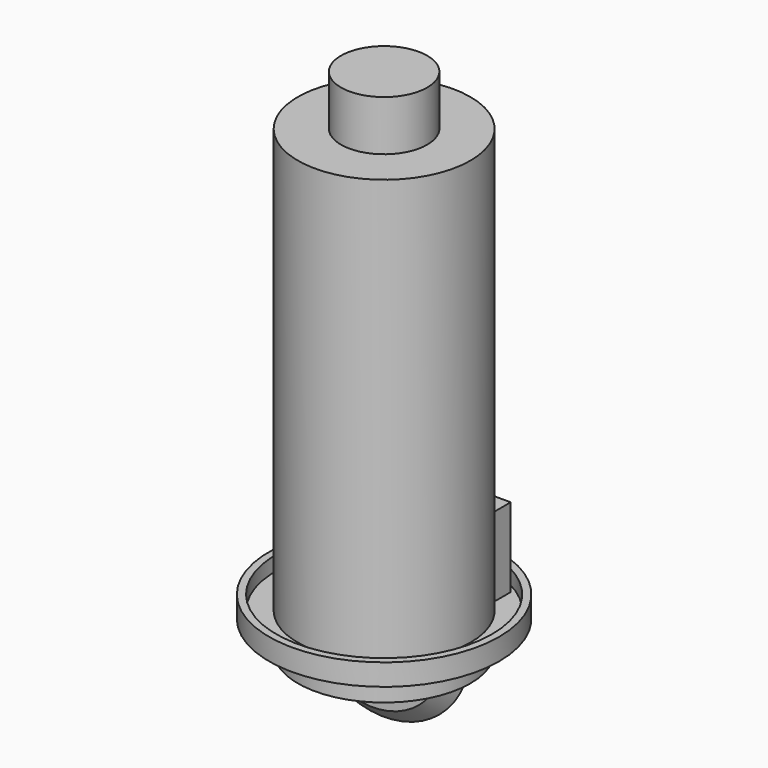
from build123d import *

# Parameters (mm, degrees)
F1_DEPTH  = 76.2
F2_R      = 76.2
F3_DEPTH  = 12.7
F4_SIZE   = 12.69999
F5_R      = 76.2
F5_R_2    = 69.85
F6_DEPTH  = 355.6
F7_R      = 76.2
F8_DEPTH  = 25.4
F9_R      = 76.2
F9_R_2    = 38.1
F10_DEPTH = 25.4
F11_R     = 101.6
F12_DEPTH = 6.35
F13_R     = 101.6
F13_R_2   = 95.25
F14_DEPTH = 12.7
F15_R     = 73.025
F16_DEPTH = 63.5
F17_R     = 38.1
F18_DEPTH = 361.95


# Not quite as in the source:
# - a fillet or chamfer is up to 0.001 mm smaller than in the source, because OpenCascade refuses the exact size


with BuildPart() as f1:
    # F0 (on Top) → F1 (new body)
    with BuildSketch(Plane.XY):
        with BuildLine():
            Line((-25.4, 0), (-50.8, 0))
            ThreePointArc((-50.8, 0), (0, -50.8), (50.8, 0))
            Line((50.8, 0), (25.4, 0))
            ThreePointArc((25.4, 0), (0, -25.4), (-25.4, 0))
        make_face()
        with BuildLine():
            Line((-50.8, 76.2), (-50.8, 0))
            Line((-50.8, 0), (-25.4, 0))
            ThreePointArc((-25.4, 0), (0, 25.4), (25.4, 0))
            Line((25.4, 0), (50.8, 0))
            Line((50.8, 0), (50.8, 76.2))
            Line((50.8, 76.2), (-50.8, 76.2))
        make_face()
    extrude(amount=F1_DEPTH)


with BuildPart() as f3:
    # F2 (on Front) → F3 (new body)
    with BuildSketch(Plane.XZ):
        Circle(F2_R)
    extrude(amount=F3_DEPTH)

    # F4 (size 12.7 in the source; OpenCascade refuses exactly that, so slightly less here)
    f4_edges = [f3.edges().sort_by_distance(p)[0] for p in [
        (-76.2, -12.7, 0),
    ]]
    chamfer(f4_edges, length=F4_SIZE)


with BuildPart() as f6:
    # F5 (on Top) → F6 (new body)
    with BuildSketch(Plane.XY):
        Circle(F5_R)
        Circle(F5_R_2, mode=Mode.SUBTRACT)
    extrude(amount=F6_DEPTH)

    # F7 (on face) → F8 (join)
    with BuildSketch(Plane(origin=(0, 0, 0), x_dir=(1, 0, 0), z_dir=(0, 0, -1))):
        Circle(F7_R)
    extrude(amount=F8_DEPTH)

    # F9 (on face) → F10 (join)
    with BuildSketch(Plane.XY.offset(355.6)):
        Circle(F9_R)
        Circle(F9_R_2, mode=Mode.SUBTRACT)
    extrude(amount=F10_DEPTH)


with BuildPart() as f12:
    # F11 (on Top) → F12 (new body)
    with BuildSketch(Plane.XY):
        Circle(F11_R)
    extrude(amount=F12_DEPTH)

    # F13 (on face) → F14 (join)
    with BuildSketch(Plane.XY.offset(6.35)):
        Circle(F13_R)
        Circle(F13_R_2, mode=Mode.SUBTRACT)
    extrude(amount=F14_DEPTH)


with BuildPart() as f16:
    # F15 (on Top) → F16 (new body)
    with BuildSketch(Plane.XY):
        Circle(F15_R)
    extrude(amount=F16_DEPTH)

    # F17 (on face) → F18 (join)
    with BuildSketch(Plane.XY.offset(63.5)):
        Circle(F17_R)
    extrude(amount=F18_DEPTH)


solid = Compound([f1.part, f3.part, f6.part, f12.part, f16.part])
